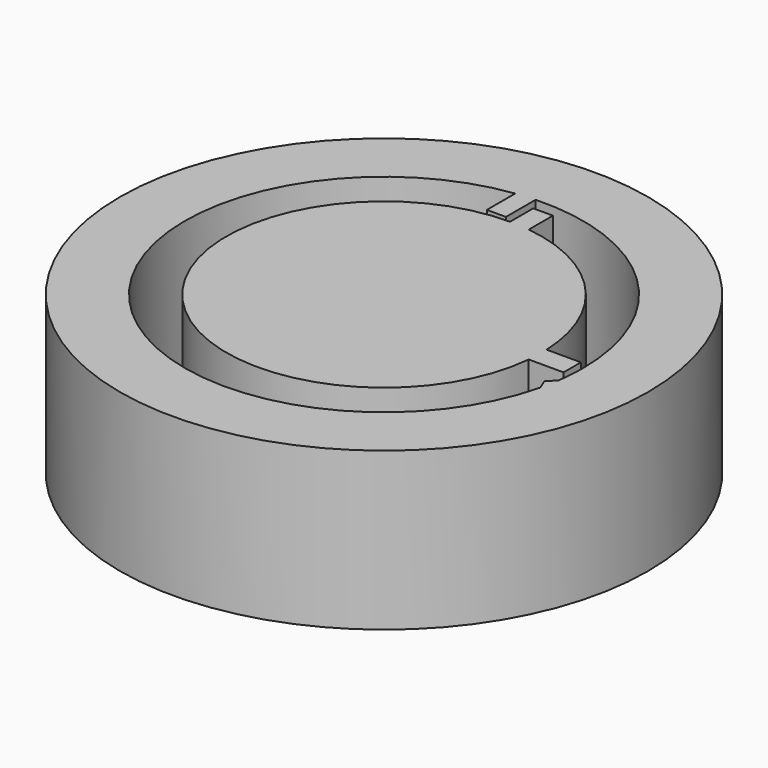
from build123d import *

# Parameters (mm, degrees)
F1_DEPTH = 25
F0_R     = 41.9000014663
F2_DEPTH = 25


# Not quite as in the source:
# - a feature names something its author has since deleted; it is built from what else it names


with BuildPart() as f1:
    # F0 (on Top) → F1 (new body)
    with BuildSketch(Plane.XY):
        with BuildLine():
            ThreePointArc((24.978908438, 1.0267099133), (24.9947265533, 0.5134632655), (25, 0))
            ThreePointArc((25, 0), (24.9707623545, -1.2087296779), (24.8831178053, -2.414632123))
            Line((24.8831178053, -2.414632123), (30.4177384824, -2.414632123))
            Line((30.4177384824, -2.414632123), (30.4177384824, 1.0267099133))
            Line((30.4177384824, 1.0267099133), (24.978908438, 1.0267099133))
        make_face()
        with BuildLine():
            Line((23.4767496586, 1.0267099133), (24.978908438, 1.0267099133))
            ThreePointArc((24.978908438, 1.0267099133), (18.4053000445, 16.9187744908), (3.1217134092, 24.8043323916))
            Line((3.1217134092, 24.8043323916), (3.1217134092, 22.8428095579))
            Line((3.1217134092, 22.8428095579), (0, 22.8428095579))
            Line((0, 22.8428095579), (0, 25))
            ThreePointArc((0, 25), (-18.5116963441, -16.8022944404), (24.8831178053, -2.414632123))
            Line((24.8831178053, -2.414632123), (23.4767496586, -2.414632123))
            Line((23.4767496586, -2.414632123), (23.4767496586, 1.0267099133))
        make_face()
        with BuildLine():
            ThreePointArc((24.8831178053, -2.414632123), (24.9707623545, -1.2087296779), (25, 0))
            ThreePointArc((25, 0), (24.9947265533, 0.5134632655), (24.978908438, 1.0267099133))
            Line((24.978908438, 1.0267099133), (23.4767496586, 1.0267099133))
            Line((23.4767496586, 1.0267099133), (23.4767496586, -2.414632123))
            Line((23.4767496586, -2.414632123), (24.8831178053, -2.414632123))
        make_face()
        with BuildLine():
            Line((3.1217134092, 22.8428095579), (3.1217134092, 24.8043323916))
            ThreePointArc((3.1217134092, 24.8043323916), (1.5639197887, 24.9510351468), (0, 25))
            Line((0, 25), (0, 22.8428095579))
            Line((0, 22.8428095579), (3.1217134092, 22.8428095579))
        make_face()
        with BuildLine():
            ThreePointArc((0, 25), (1.5639197887, 24.9510351468), (3.1217134092, 24.8043323916))
            Line((3.1217134092, 24.8043323916), (3.1217134092, 29.5925959945))
            Line((3.1217134092, 29.5925959945), (0, 29.5925959945))
            Line((0, 29.5925959945), (0, 25))
        make_face()
    extrude(amount=F1_DEPTH)


with BuildPart() as f2:
    # F0 (on Top) → F2 (new body)
    with BuildSketch(Plane.XY):
        Circle(F0_R)
        with BuildLine():
            ThreePointArc((31.2779555005, -4.4999336962), (31.0328144506, -5.9602290926), (30.7195340658, -7.4074375018))
            ThreePointArc((30.7195340658, -7.4074375018), (-23.4572255231, -21.1735324006), (-4.2332089506, 31.3151695755))
            Line((-4.2332089506, 31.3151695755), (-4.2332089506, 32.823305577))
            Line((-4.2332089506, 32.823305577), (-1.2088371441, 32.823305577))
            Line((-1.2088371441, 32.823305577), (-1.2088371441, 31.5768683742))
            ThreePointArc((-1.2088371441, 31.5768683742), (21.9130172689, 22.7679506705), (31.5999984741, 0))
            ThreePointArc((31.5999984741, 0), (31.5193849056, -2.255721334), (31.2779555005, -4.4999336962))
        make_face(mode=Mode.SUBTRACT)
        with BuildLine():
            Line((-4.2332089506, 32.823305577), (-4.2332089506, 31.3151695755))
            ThreePointArc((-4.2332089506, 31.3151695755), (-2.7241673938, 31.4823572112), (-1.2088371441, 31.5768683742))
            Line((-1.2088371441, 31.5768683742), (-1.2088371441, 32.823305577))
            Line((-1.2088371441, 32.823305577), (-4.2332089506, 32.823305577))
        make_face()
        with BuildLine():
            ThreePointArc((-1.2088371441, 31.5768683742), (-2.7241673938, 31.4823572112), (-4.2332089506, 31.3151695755))
            Line((-4.2332089506, 31.3151695755), (-4.2332089506, 25.6888903677))
            Line((-4.2332089506, 25.6888903677), (-1.2088371441, 25.6888903677))
            Line((-1.2088371441, 25.6888903677), (-1.2088371441, 31.5768683742))
        make_face()
        with BuildLine():
            Line((30.0426278263, -5.7433205657), (30.7195340658, -7.4074375018))
            ThreePointArc((30.7195340658, -7.4074375018), (31.0328144506, -5.9602290926), (31.2779555005, -4.4999336962))
            Line((31.2779555005, -4.4999336962), (30.0426278263, -5.7433205657))
        make_face()
    extrude(amount=F2_DEPTH)


solid = Compound([f1.part, f2.part])
